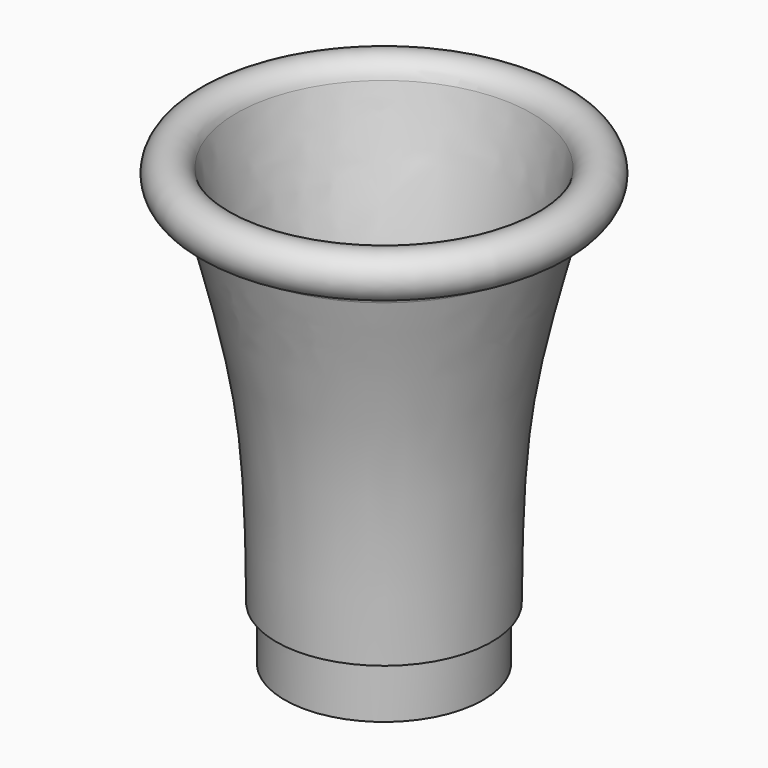
from build123d import *

# Parameters (mm, degrees)
F2_R     = 22.5
F2_R_2   = 18.5
F3_DEPTH = 10


# Not quite as in the source:
# - ends of sketch curves that miss each other by under 0.0002 mm in the source are joined
# - the dataset's text gives a spline's control points without its knots; the knots are read off the source's solid


with BuildPart() as f1:
    # F0 (on Right) → F1 (revolve)
    with BuildSketch(Plane.YZ):
        with BuildLine():
            Line((-19.999918566, -0.0221042413), (-17, 0))
            add(Edge.make_bspline(
                [(-17, 0), (-17.1100714453, 14.9385526751), (-16.6501725085, 43.9371220907), (-24.7594404053, 69.4739705275), (-27.5, 81.2049582601)],
                knots=[0, 0, 0, 0, 0.5182501459, 1, 1, 1, 1], degree=3))
            ThreePointArc((-27.5, 81.2049582601), (-34.4680485067, 82.8556771544), (-31.5876355337, 76.2996269742))
            ThreePointArc((-31.5876355337, 76.2996269742), (-29.8360350078, 75.6280192423), (-28.8257994316, 74.0473278023))
            add(Edge.make_bspline(
                [(-19.999918566, -0.0221042413), (-20.0265504384, 3.5922902833), (-20.0391016699, 10.8108769326), (-20.1590781414, 21.5220738722), (-20.5260867717, 30.2770305254), (-21.0871523738, 37.1325499921), (-21.5708100593, 41.3470099171), (-22.0510428697, 44.6683392237), (-22.5959202299, 47.9702777058), (-23.3839580199, 52.0623829172), (-24.4623113385, 56.9196909992), (-26.0240091098, 63.3294255046), (-27.5282289103, 69.0264613417), (-28.5832353261, 73.1000377108), (-28.8257994316, 74.0473278023)],
                knots=[0, 0, 0, 0, 0.125, 0.25, 0.375, 0.4375, 0.5, 0.53125, 0.5625, 0.625, 0.6875, 0.75, 0.875, 0.9129922864, 0.9129922864, 0.9129922864, 0.9129922864], degree=3))
        make_face()
    revolve(axis=Axis((0, 0, 40.60247913), (0, 0, 1)))

    # F2 (on Top) → F3 (cut, symmetric)
    with BuildSketch(Plane.XY):
        Circle(F2_R)
        Circle(F2_R_2, mode=Mode.SUBTRACT)
    extrude(amount=F3_DEPTH, both=True, mode=Mode.SUBTRACT)


solid = f1.part
